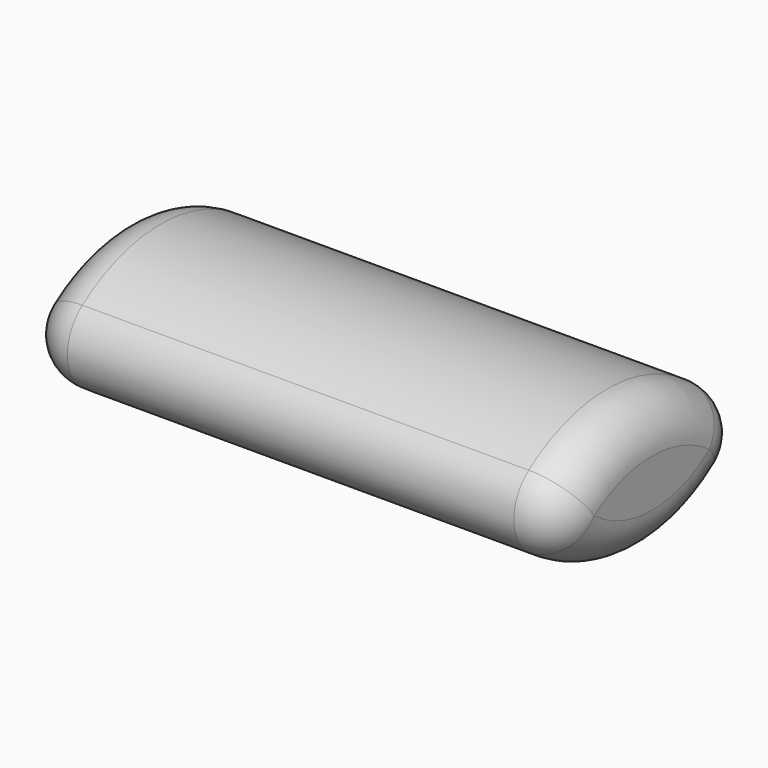
from build123d import *

# Parameters (mm, degrees)
F1_DEPTH = 600
F3_R     = 50


# Not quite as in the source:
# - a feature of the source that left no trace in its solid (it failed there, or was rolled back) is left out


with BuildPart() as f1:
    # F0 (on Right) → F1 (new body)
    with BuildSketch(Plane.YZ):
        with BuildLine():
            ThreePointArc((0, 0), (150, -78.7228552032), (300, 0))
            ThreePointArc((300, 0), (150, 74.7485079271), (0, 0))
        make_face()
    extrude(amount=F1_DEPTH)

    # F3
    f3_edges = [f1.edges().sort_by_distance(p)[0] for p in [
        (600, 150, 74.748508),
        (600, 150, -78.722855),
        (0, 150, 74.748508),
        (0, 150, -78.722855),
        (300, 300, 0),
        (300, 0, 0),
    ]]
    fillet(f3_edges, radius=F3_R)


solid = f1.part
